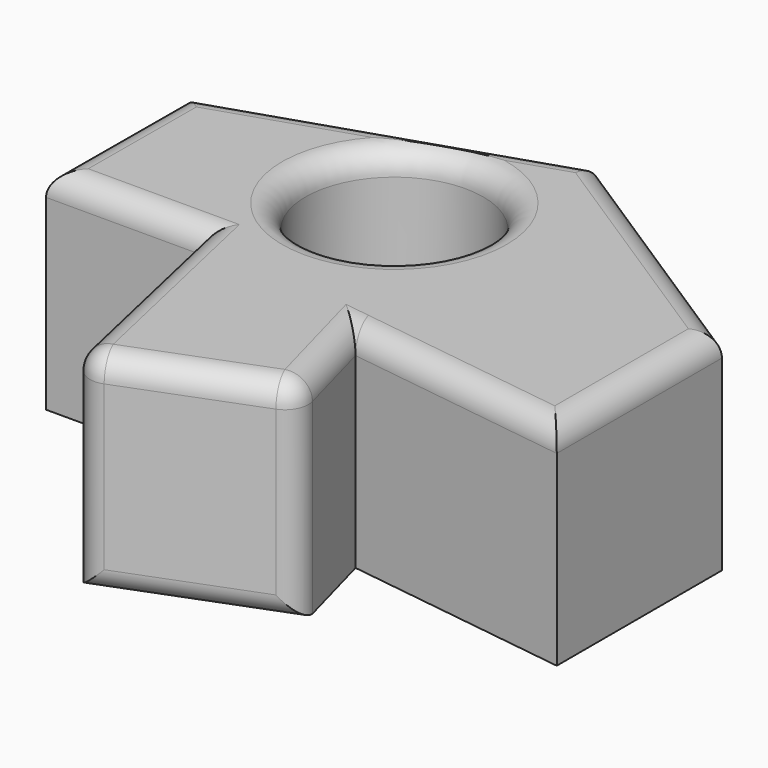
from build123d import *

# Parameters (mm, degrees)
F0_R         = 19.3201303499
F1_DEPTH     = 45.72
F2_T1_DEPTH  = 55.325963316
F2_T3_DEPTH  = 52.1146440054
F2_T5_DEPTH  = 66.4513256331
F2_T7_DEPTH  = 30.5870827045
F2_T9_DEPTH  = 100.2395855595
F2_T11_DEPTH = 63.3652483976
F2_T13_DEPTH = 70.2836609721
F2_T15_DEPTH = 91.0933305156
F2_T20_DEPTH = 5.08
F2_T26_DEPTH = 5.08
F2_T36_DEPTH = 59.2845010847
F2_T41_DEPTH = 57.568004282
F2_T46_DEPTH = 31.0915483116
F2_T51_DEPTH = 75.0016446771
F2_T57_DEPTH = 59.2845010847
F2_T61_DEPTH = 57.568004282
F2_T68_DEPTH = 31.0915483116
F2_T72_DEPTH = 75.0016446771


# Not quite as in the source:
# - a fillet or chamfer that OpenCascade refuses, or shapes differently, is made with other operations: its cross-section is extruded or revolved along the edge and cut away or added


with BuildPart() as f1:
    # F0 (on Top) → F1 (new body)
    with BuildSketch(Plane.XY):
        Polygon((13.1280273199, 53.9313554764), (-58.0116845667, 30.691197142), (-58.1890903413, -7.2736367583), (-24.3045892566, -7.2736367583), (-13.1280263886, -56.7698441446), (25.1916181296, -42.0451648533), (19.1598236561, -19.8694467545), (68.3012157679, -26.610866189), (68.3012157679, 18.2727947831), align=None)
        with Locations((-4.6125496738, 20.4016622156)):
            Circle(F0_R, mode=Mode.SUBTRACT)
    extrude(amount=F1_DEPTH)

    # F2: fillet of radius 5.08 on 15 edges, made by hand

    # F2_s2 → F2_t1 (cut)
    with BuildSketch(Plane.XY.offset(-14.685963316)):
        with BuildLine():
            ThreePointArc((-14.4219236098, -51.039727833), (-11.8616097658, -54.4008391443), (-7.6445406789, -54.662763834))
            Line((-7.6445406789, -54.662763834), (-13.1280263886, -56.7698441446))
            Line((-13.1280263886, -56.7698441446), (-14.4219236098, -51.039727833))
        make_face()
    extrude(amount=F2_T1_DEPTH, mode=Mode.SUBTRACT)

    # F2_s4 → F2_t3 (cut)
    with BuildSketch(Plane.XY.offset(-11.4746440054)):
        with BuildLine():
            ThreePointArc((20.9071837297, -43.6914985622), (23.6160955732, -41.2464799373), (23.9869451943, -37.6162196147))
            Line((23.9869451943, -37.6162196147), (25.1916181296, -42.0451648533))
            Line((25.1916181296, -42.0451648533), (20.9071837297, -43.6914985622))
        make_face()
    extrude(amount=F2_T3_DEPTH, mode=Mode.SUBTRACT)

    # F2_s6 → F2_t5 (cut)
    with BuildSketch(Plane(origin=(-42.3016489373, -16.2548014713, 0), x_dir=(0, 0, 1), z_dir=(0.9334569329, 0.3586894958, 0))):
        with BuildLine():
            ThreePointArc((5.08, 48.2833194327), (1.4878975516, 46.7954218811), (0, 43.2033194327))
            Line((0, 43.2033194327), (0, 48.2833194327))
            Line((0, 48.2833194327), (5.08, 48.2833194327))
        make_face()
    extrude(amount=F2_T5_DEPTH, mode=Mode.SUBTRACT)

    # F2_s8 → F2_t7 (cut)
    with BuildSketch(Plane(origin=(-24.9632601794, -9.5923645646, 0), x_dir=(0, 0, 1), z_dir=(0.9334569329, 0.3586894958, 0))):
        with BuildLine():
            ThreePointArc((40.64, 48.2833194327), (44.2321024484, 46.7954218811), (45.72, 43.2033194327))
            Line((45.72, 43.2033194327), (45.72, 48.2833194327))
            Line((45.72, 48.2833194327), (40.64, 48.2833194327))
        make_face()
    extrude(amount=F2_T7_DEPTH, mode=Mode.SUBTRACT)

    # F2_s10 → F2_t9 (cut)
    with BuildSketch(Plane(origin=(39.8537401384, 13.0195527431, 0), x_dir=(0, 0, 1), z_dir=(-0.9505626114, -0.3105329641, 0))):
        with BuildLine():
            ThreePointArc((40.64, 47.1884448626), (44.2321024484, 45.700547311), (45.72, 42.1084448626))
            Line((45.72, 42.1084448626), (45.72, 47.1884448626))
            Line((45.72, 47.1884448626), (40.64, 47.1884448626))
        make_face()
    extrude(amount=F2_T9_DEPTH, mode=Mode.SUBTRACT)

    # F2_s12 → F2_t11 (cut)
    with BuildSketch(Plane(origin=(0.2014921201, 43.1193115962, 0), x_dir=(0, 0, 1), z_dir=(-0.0046728464, -0.9999890822, 0))):
        with BuildLine():
            ThreePointArc((40.64, 58.1544664567), (44.2321024484, 56.6665689051), (45.72, 53.0744664567))
            Line((45.72, 53.0744664567), (45.72, 58.1544664567))
            Line((45.72, 58.1544664567), (40.64, 58.1544664567))
        make_face()
    extrude(amount=F2_T11_DEPTH, mode=Mode.SUBTRACT)

    # F2_s14 → F2_t13 (cut)
    with BuildSketch(Plane.XZ.offset(-30.9727947831)):
        with BuildLine():
            ThreePointArc((68.3012157679, 40.64), (66.8133182163, 44.2321024484), (63.2212157679, 45.72))
            Line((63.2212157679, 45.72), (68.3012157679, 45.72))
            Line((68.3012157679, 45.72), (68.3012157679, 40.64))
        make_face()
    extrude(amount=F2_T13_DEPTH, mode=Mode.SUBTRACT)

    # F2_s16 → F2_t15 (cut)
    with BuildSketch(Plane(origin=(50.5132947185, -32.6468604807, 0), x_dir=(0, 0, 1), z_dir=(-0.8398598155, 0.5428033624, 0))):
        with BuildLine():
            ThreePointArc((40.64, 52.4207156327), (44.2321024484, 50.9328180811), (45.72, 47.3407156327))
            Line((45.72, 47.3407156327), (45.72, 52.4207156327))
            Line((45.72, 52.4207156327), (40.64, 52.4207156327))
        make_face()
    extrude(amount=F2_T15_DEPTH, mode=Mode.SUBTRACT)


with BuildPart() as f2_tool18:
    # F2_s19 → F2_t20 (new body)
    with BuildSketch(Plane.XY.offset(40.64)):
        Polygon((-9.4666833174, -49.9208026147), (-14.4219236098, -51.039727833), (-13.1280263886, -56.7698441446), (-7.6445406789, -54.662763834), align=None)
    extrude(amount=F2_T20_DEPTH)

    # F2_s21 → F2_t22 (revolve, cut)
    with BuildSketch(Plane(origin=(-9.4666833174, -49.9208026147, 40.64), x_dir=(0.4714422143, 0.8818969546, 0), z_dir=(0.8818969546, -0.4714422143, 0))):
        with BuildLine():
            ThreePointArc((0, -5.08), (5.08, 0), (0, 5.08))
            Line((0, 5.08), (0, -5.08))
        make_face()
    revolve(axis=Axis((-9.4666833174, -49.9208026147, 40.64), (0, 0, 1)), mode=Mode.SUBTRACT)


with BuildPart() as f1_1:
    add(f1.part)

    # F2_t17: cut F2_tool18
    add(f2_tool18.part, mode=Mode.SUBTRACT)


with BuildPart() as f2_tool24:
    # F2_s25 → F2_t26 (new body)
    with BuildSketch(Plane.XY.offset(40.64)):
        Polygon((19.0850410913, -38.9495373429), (20.9071837297, -43.6914985622), (25.1916181296, -42.0451648533), (23.9869451943, -37.6162196147), align=None)
    extrude(amount=F2_T26_DEPTH)

    # F2_s27 → F2_t28 (revolve, cut)
    with BuildSketch(Plane(origin=(19.0850410913, -38.9495373429, 40.64), x_dir=(-0.8919398586, 0.452154054, 0), z_dir=(0.452154054, 0.8919398586, 0))):
        with BuildLine():
            ThreePointArc((0, -5.08), (5.08, 0), (0, 5.08))
            Line((0, 5.08), (0, -5.08))
        make_face()
    revolve(axis=Axis((19.0850410913, -38.9495373429, 40.64), (0, 0, 1)), mode=Mode.SUBTRACT)


with BuildPart() as f1_2:
    add(f1_1.part)

    # F2_t23: cut F2_tool24
    add(f2_tool24.part, mode=Mode.SUBTRACT)

    # F2_s29 → F2_t30 (revolve, cut)
    with BuildSketch(Plane.XZ.offset(-20.4016622156)):
        with BuildLine():
            ThreePointArc((14.7075806761, 5.08), (16.1954782277, 1.4878975516), (19.7875806761, 0))
            Line((19.7875806761, 0), (14.7075806761, 0))
            Line((14.7075806761, 0), (14.7075806761, 5.08))
        make_face()
    revolve(axis=Axis((-4.6125496738, 20.4016622156, 0), (0, 0, 1)), mode=Mode.SUBTRACT)

    # F2_s31 → F2_t32 (revolve, cut)
    with BuildSketch(Plane.XZ.offset(-20.4016622156)):
        with BuildLine():
            ThreePointArc((14.7075806761, 40.64), (16.1954782277, 44.2321024484), (19.7875806761, 45.72))
            Line((19.7875806761, 45.72), (14.7075806761, 45.72))
            Line((14.7075806761, 45.72), (14.7075806761, 40.64))
        make_face()
    revolve(axis=Axis((-4.6125496738, 20.4016622156, 45.72), (0, 0, 1)), mode=Mode.SUBTRACT)


with BuildPart() as f2_tool34:
    # F2_s35 → F2_t36 (new body)
    with BuildSketch(Plane.YZ.offset(-70.8890903413)):
        with BuildLine():
            ThreePointArc((-7.2736367583, 40.64), (-5.7857392068, 44.2321024484), (-2.1936367583, 45.72))
            Line((-2.1936367583, 45.72), (-7.2736367583, 45.72))
            Line((-7.2736367583, 45.72), (-7.2736367583, 40.64))
        make_face()
    extrude(amount=F2_T36_DEPTH)

    split(bisect_by=Plane(origin=(-24.6882073851, -5.5747564614, 0), x_dir=(0, 0, 1), z_dir=(-0.9754410024, -0.2202608697, 0)), keep=Keep.TOP)


with BuildPart() as f1_3:
    add(f1_2.part)

    # F2_t33: cut F2_tool34
    add(f2_tool34.part, mode=Mode.SUBTRACT)


with BuildPart() as f2_tool39:
    # F2_s40 → F2_t41 (new body)
    with BuildSketch(Plane(origin=(-2.4136949173, 10.6892204341, 0), x_dir=(0, 0, 1), z_dir=(0.2202608697, -0.9754410024, 0))):
        with BuildLine():
            ThreePointArc((40.64, 25.3097904672), (44.2321024484, 23.8218929156), (45.72, 20.2297904672))
            Line((45.72, 20.2297904672), (45.72, 25.3097904672))
            Line((45.72, 25.3097904672), (40.64, 25.3097904672))
        make_face()
    extrude(amount=F2_T41_DEPTH)

    split(bisect_by=Plane.XZ.offset(7.2736367583), keep=Keep.TOP)


with BuildPart() as f1_4:
    add(f1_3.part)

    # F2_t38: cut F2_tool39
    add(f2_tool39.part, mode=Mode.SUBTRACT)


with BuildPart() as f2_tool44:
    # F2_s45 → F2_t46 (new body)
    with BuildSketch(Plane(origin=(11.1791797465, -41.0999313259, 0), x_dir=(0, 0, 1), z_dir=(-0.2624641197, 0.9649417526, 0))):
        with BuildLine():
            ThreePointArc((40.64, 13.2730969655), (44.2321024484, 11.7851994139), (45.72, 8.1930969655))
            Line((45.72, 8.1930969655), (45.72, 13.2730969655))
            Line((45.72, 13.2730969655), (40.64, 13.2730969655))
        make_face()
    extrude(amount=F2_T46_DEPTH)

    split(bisect_by=Plane(origin=(-2.3215052957, -16.9225491951, 0), x_dir=(0, 0, 1), z_dir=(-0.1359112078, -0.9907210221, 0)), keep=Keep.TOP)


with BuildPart() as f1_5:
    add(f1_4.part)

    # F2_t43: cut F2_tool44
    add(f2_tool44.part, mode=Mode.SUBTRACT)


with BuildPart() as f2_tool49:
    # F2_s50 → F2_t51 (new body)
    with BuildSketch(Plane(origin=(8.8991719713, -1.2208252209, 0), x_dir=(0, 0, 1), z_dir=(0.9907210221, -0.1359112078, 0))):
        with BuildLine():
            ThreePointArc((40.64, 17.0810438235), (44.2321024484, 15.5931462719), (45.72, 12.0010438235))
            Line((45.72, 12.0010438235), (45.72, 17.0810438235))
            Line((45.72, 17.0810438235), (40.64, 17.0810438235))
        make_face()
    extrude(amount=F2_T51_DEPTH)

    split(bisect_by=Plane(origin=(12.8077654479, 3.4837117113, 0), x_dir=(0, 0, 1), z_dir=(0.9649417526, 0.2624641197, 0)), keep=Keep.TOP)


with BuildPart() as f1_6:
    add(f1_5.part)

    # F2_t48: cut F2_tool49
    add(f2_tool49.part, mode=Mode.SUBTRACT)


with BuildPart() as f2_tool55:
    # F2_s56 → F2_t57 (new body)
    with BuildSketch(Plane.YZ.offset(-70.8890903413)):
        with BuildLine():
            ThreePointArc((-7.2736367583, 40.64), (-5.7857392068, 44.2321024484), (-2.1936367583, 45.72))
            Line((-2.1936367583, 45.72), (-7.2736367583, 45.72))
            Line((-7.2736367583, 45.72), (-7.2736367583, 40.64))
        make_face()
    extrude(amount=F2_T57_DEPTH)

    split(bisect_by=Plane(origin=(-24.6882073851, -5.5747564614, 0), x_dir=(0, 0, 1), z_dir=(0.9754410024, 0.2202608697, 0)), keep=Keep.TOP)


with BuildPart() as f2_tool59:
    # F2_s60 → F2_t61 (new body)
    with BuildSketch(Plane(origin=(-2.4136949173, 10.6892204341, 0), x_dir=(0, 0, 1), z_dir=(0.2202608697, -0.9754410024, 0))):
        with BuildLine():
            ThreePointArc((40.64, 25.3097904672), (44.2321024484, 23.8218929156), (45.72, 20.2297904672))
            Line((45.72, 20.2297904672), (45.72, 25.3097904672))
            Line((45.72, 25.3097904672), (40.64, 25.3097904672))
        make_face()
    extrude(amount=F2_T61_DEPTH)

    split(bisect_by=Plane.XZ.offset(7.2736367583), keep=Keep.BOTTOM)


with BuildPart() as f2_tool55_1:
    add(f2_tool55.part)

    # F2_t63: intersect F2_tool59
    add(f2_tool59.part, mode=Mode.INTERSECT)


with BuildPart() as f1_7:
    add(f1_6.part)

    # F2_t53: cut F2_tool55
    add(f2_tool55_1.part, mode=Mode.SUBTRACT)


with BuildPart() as f2_tool66:
    # F2_s67 → F2_t68 (new body)
    with BuildSketch(Plane(origin=(11.1791797465, -41.0999313259, 0), x_dir=(0, 0, 1), z_dir=(-0.2624641197, 0.9649417526, 0))):
        with BuildLine():
            ThreePointArc((40.64, 13.2730969655), (44.2321024484, 11.7851994139), (45.72, 8.1930969655))
            Line((45.72, 8.1930969655), (45.72, 13.2730969655))
            Line((45.72, 13.2730969655), (40.64, 13.2730969655))
        make_face()
    extrude(amount=F2_T68_DEPTH)

    split(bisect_by=Plane(origin=(-2.3215052957, -16.9225491951, 0), x_dir=(0, 0, 1), z_dir=(0.1359112078, 0.9907210221, 0)), keep=Keep.TOP)


with BuildPart() as f2_tool70:
    # F2_s71 → F2_t72 (new body)
    with BuildSketch(Plane(origin=(8.8991719713, -1.2208252209, 0), x_dir=(0, 0, 1), z_dir=(0.9907210221, -0.1359112078, 0))):
        with BuildLine():
            ThreePointArc((40.64, 17.0810438235), (44.2321024484, 15.5931462719), (45.72, 12.0010438235))
            Line((45.72, 12.0010438235), (45.72, 17.0810438235))
            Line((45.72, 17.0810438235), (40.64, 17.0810438235))
        make_face()
    extrude(amount=F2_T72_DEPTH)

    split(bisect_by=Plane(origin=(12.8077654479, 3.4837117113, 0), x_dir=(0, 0, 1), z_dir=(-0.9649417526, -0.2624641197, 0)), keep=Keep.TOP)


with BuildPart() as f2_tool66_1:
    add(f2_tool66.part)

    # F2_t74: intersect F2_tool70
    add(f2_tool70.part, mode=Mode.INTERSECT)


with BuildPart() as f1_8:
    add(f1_7.part)

    # F2_t64: cut F2_tool66
    add(f2_tool66_1.part, mode=Mode.SUBTRACT)


solid = f1_8.part
